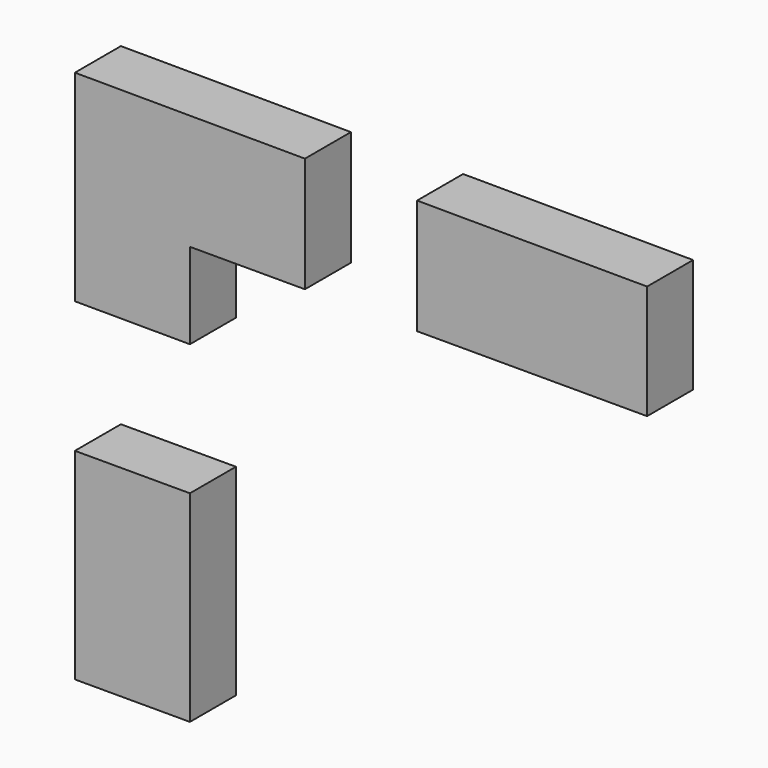
from build123d import *

# Parameters (mm, degrees)
F1_DEPTH = 25.4
F0_W     = 50.8
F0_H     = 88.9
F2_DEPTH = 25.4
F3_DEPTH = 25.4


# Not quite as in the source:
# - the program builds the solid bodies; features that only make, move or delete a surface that nothing else refers to are left out


with BuildPart() as f1:
    # F0 (on Front) → F1 (new body)
    with BuildSketch(Plane.XZ):
        Polygon((151.13, 184.5482311558), (252.73, 184.5482311558), (252.73, 234.95), (151.13, 235.3482311558), align=None)
    extrude(amount=F1_DEPTH)


with BuildPart() as f1b:
    # F0 (on Front) → F1, piece 2 (new body)
    with BuildSketch(Plane.XZ):
        Polygon((51.1480593626, 235.7401201693), (50.9481686791, 184.7423688442), (101.6, 184.7423688442), (101.6, 235.5423688442), align=None)
    extrude(amount=F1_DEPTH)

    # F0 (on Front) → F3 (join)
    with BuildSketch(Plane.XZ):
        Polygon((0, 235.9406), (0, 184.7423688442), (50.9481686791, 184.7423688442), (51.1480593626, 235.7401201693), align=None)
        Polygon((0, 184.7423688442), (0, 147.0399171062), (50.799609778, 146.8408030579), (50.9481686791, 184.7423688442), align=None)
    extrude(amount=F3_DEPTH)


with BuildPart() as f2:
    # F0 (on Front) → F2 (new body)
    with BuildSketch(Plane.XZ):
        with Locations((25.4, 44.45)):
            Rectangle(F0_W, F0_H)
    extrude(amount=F2_DEPTH)


solid = Compound([f1.part, f1b.part, f2.part])
